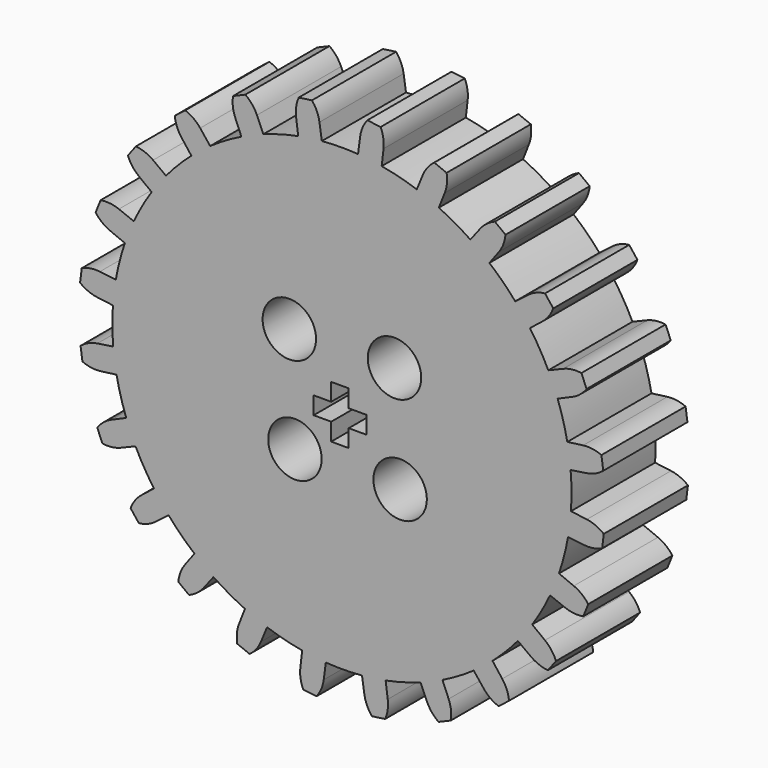
from build123d import *

# Parameters (mm, degrees)
F2_R            = 17.46
F2_R_2          = 2.0320626532
F3_DEPTH        = 8
F4_DEPTH        = 8
F4_COPIES_COUNT = 24
F6_DEPTH        = 25.4


# Not quite as in the source:
# - a pattern or mirror of a feature is missing from the dataset's text; its kind, count and spacing are read off the source's solid


with BuildPart() as f3:
    # F2 (on Front) → F3 (new body)
    with BuildSketch(Plane.XZ):
        Circle(F2_R)
        with Locations((-3.5724579239, -3.8998227125)):
            Circle(F2_R_2, mode=Mode.SUBTRACT)
        with Locations((4.4270495434, -3.9885936614)):
            Circle(F2_R_2, mode=Mode.SUBTRACT)
        with Locations((-4, 4)):
            Circle(F2_R_2, mode=Mode.SUBTRACT)
        with Locations((4, 4)):
            Circle(F2_R_2, mode=Mode.SUBTRACT)
    extrude(amount=F3_DEPTH)

    # F0 (on Front) → F4 (join, through all)
    with BuildSketch(Plane.XZ):
        with BuildLine():
            Line((2.9415938455, 19.7890142005), (1.9331669555, 19.9128334534))
            ThreePointArc((1.9331669555, 19.9128334534), (1.5696265728, 19.3072255779), (1.3834076243, 18.6258703021))
            Line((1.3834076243, 18.6258703021), (1.2255142043, 17.4169375877))
            ThreePointArc((1.2255142043, 17.4169375877), (2.1278274415, 17.3298571944), (3.0244049475, 17.1960627678))
            Line((3.0244049475, 17.1960627678), (3.1636731251, 18.4072824071))
            ThreePointArc((3.1636731251, 18.4072824071), (3.1478229298, 19.1134476574), (2.9415938455, 19.7890142005))
        make_face()
    f4 = extrude(amount=F4_DEPTH)

    # F4_copies: F4 ×24 about axis
    f4_copies_axis = Axis((0, 0, 0), (0, 1, 0))
    for i in range(1, F4_COPIES_COUNT):
        add(f4.rotate(f4_copies_axis, i * 360 / F4_COPIES_COUNT))

    # F5 (on Front) → F6 (cut)
    with BuildSketch(Plane.XZ):
        Polygon((0.5182245299, 0.1698074956), (0.5182245299, 1.503140829), (-0.1484421367, 1.503140829), (-0.8151088034, 1.503140829), (-0.8151088034, 0.1698074956), (-2.1484421367, 0.1698074956), (-2.1484421367, -0.496859171), (-2.1484421367, -1.1635258377), (-0.8151088034, -1.1635258377), (-0.8151088034, -2.496859171), (-0.1484421367, -2.496859171), (0.5182245299, -2.496859171), (0.5182245299, -1.1635258377), (1.8515578633, -1.1635258377), (1.8515578633, -0.496859171), (1.8515578633, 0.1698074956), align=None)
    extrude(amount=F6_DEPTH, mode=Mode.SUBTRACT)


solid = f3.part
